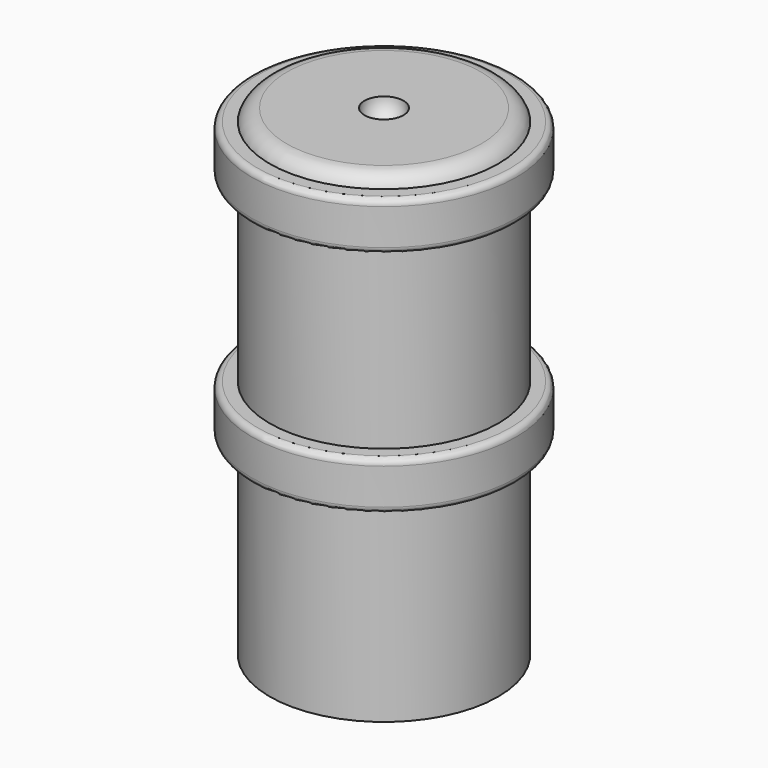
from build123d import *


# Not quite as in the source:
# - a fillet or chamfer that OpenCascade refuses, or shapes differently, is made with other operations: its cross-section is extruded or revolved along the edge and cut away or added


with BuildPart() as f1:
    # F0 (on Front) → F1 (revolve)
    with BuildSketch(Plane.XZ):
        with BuildLine():
            Line((9.5, 20), (1.625, 20))
            ThreePointArc((1.625, 20), (1.1490485194, 18.8509514806), (0, 18.375))
            Line((0, 18.375), (0, 17.5))
            Line((0, 17.5), (8.2, 17.5))
            Line((8.2, 17.5), (8.3229769486, 7.2519209513))
            ThreePointArc((8.3229769486, 7.2519209513), (8.2000935899, 6.6844011231), (8.3365600781, 6.1199934931))
            Line((8.3365600781, 6.1199934931), (8.65, -20))
            Line((8.65, -20), (9.5, -20))
            Line((9.5, -20), (9.5, -4))
            Line((9.5, -4), (10.5, -4))
            ThreePointArc((10.5, -4), (10.8535533906, -3.8535533906), (11, -3.5))
            Line((11, -3.5), (11, -0.5))
            ThreePointArc((11, -0.5), (10.8535533906, -0.1464466094), (10.5, 0))
            Line((10.5, 0), (9.5, 0))
            Line((9.5, 0), (9.5, 15))
            Line((9.5, 15), (10.5, 15))
            ThreePointArc((10.5, 15), (10.8535533906, 15.1464466094), (11, 15.5))
            Line((11, 15.5), (11, 18.5))
            ThreePointArc((11, 18.5), (10.8535533906, 18.8535533906), (10.5, 19))
            Line((10.5, 19), (9.5, 19))
            Line((9.5, 19), (9.5, 20))
        make_face()
    revolve(axis=Axis((0, 0, 0), (0, 0, -1)))

    # F2: fillet of radius 1.5 on 1 edges, made by hand

    # F2_s1 → F2_t2 (revolve, cut)
    with BuildSketch(Plane.XZ):
        with BuildLine():
            ThreePointArc((9.5, 19), (8.9518118414, 19.7247448714), (8.0857864376, 20))
            Line((8.0857864376, 20), (9.5, 20))
            Line((9.5, 20), (9.5, 19))
        make_face()
    revolve(axis=Axis((0, 0, 20), (0, 0, -1)), mode=Mode.SUBTRACT)


solid = f1.part
